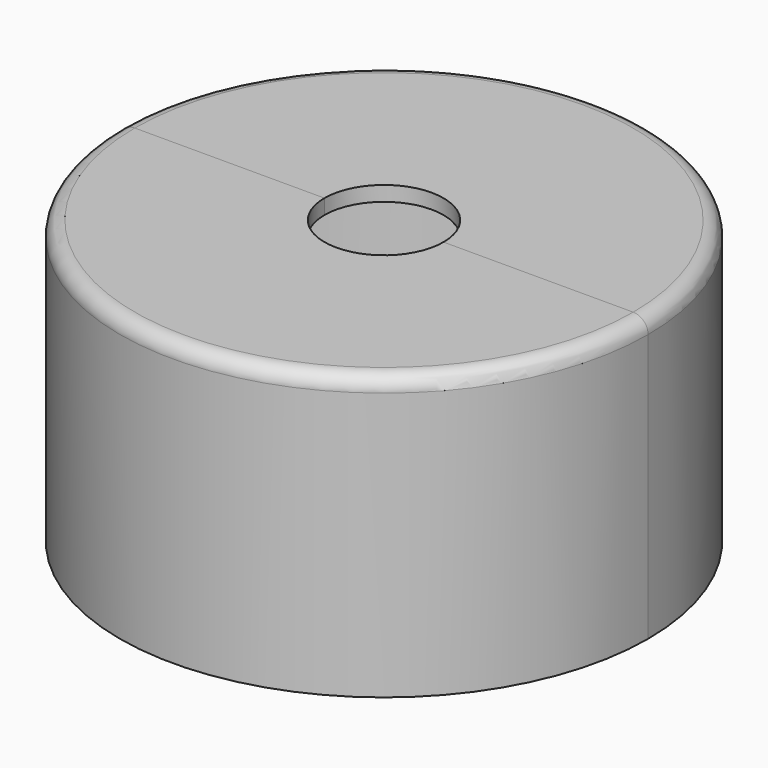
from build123d import *
from build123d import SkipClean  # not in build123d's __all__

# Parameters (mm, degrees)
F3_DEPTH  = 36
F5_DEPTH  = 20
F7_DEPTH  = 36.001
F10_R     = 10
F11_DEPTH = 7
F12_R     = 10
F12_R_2   = 8
F13_DEPTH = 2
F14_W     = 113.5210208595
F14_H     = 51.0865971446
F15_DEPTH = 38.001
F16_W     = 26.7383140922
F16_H     = 24.3122323528
F17_DEPTH = 36
F18_R     = 2
F20_DEPTH = 5


with BuildPart() as f1:
    # F0 (on Front) → F1 (revolve)
    with BuildSketch(Plane.XZ):
        Polygon((26, -5), (27.5, -5), (27.5, 31), (0, 31), (0, 26), (26, 26), (26, 0), align=None)
    revolve(axis=Axis((0, 0, 28.5), (0, 0, 1)))

    # F2 (on face) → F3 (join, through all)
    with BuildSketch(Plane(origin=(0, 0, -5), x_dir=(1, 0, 0), z_dir=(0, 0, -1))):
        with BuildLine():
            Line((-23.5584379788, 11), (23.5584379788, 11))
            ThreePointArc((23.5584379788, 11), (0, 26), (-23.5584379788, 11))
        make_face()
        with BuildLine():
            Line((23.5584379788, -11), (-23.5584379788, -11))
            ThreePointArc((-23.5584379788, -11), (0, -26), (23.5584379788, -11))
        make_face()
    extrude(amount=-F3_DEPTH)

    # F4 (on Front) → F5 (cut, symmetric)
    with BuildSketch(Plane.XZ):
        with BuildLine():
            Line((4.5, -4.6839690926), (3.5, -1.9364916731))
            ThreePointArc((3.5, -1.9364916731), (3.4457195687, 2.0315060063), (0, 4))
            ThreePointArc((0, 4), (-3.4457195687, 2.0315060063), (-3.5, -1.9364916731))
            Line((-3.5, -1.9364916731), (-4.5, -4.6839690926))
            Line((-4.5, -4.6839690926), (-4.5, -5))
            Line((-4.5, -5), (0, -5))
            Line((0, -5), (4.5, -5))
            Line((4.5, -5), (4.5, -4.6839690926))
        make_face()
    extrude(amount=F5_DEPTH, both=True, mode=Mode.SUBTRACT)

    # F6 (on face) → F7 (cut, through all)
    with BuildSketch(Plane(origin=(0, 0, -5), x_dir=(1, 0, 0), z_dir=(0, 0, -1))):
        with BuildLine():
            Line((24.2332416321, -13), (6.5, -13))
            Line((6.5, -13), (6.5, -22))
            Line((6.5, -22), (-6.5, -22))
            Line((-6.5, -22), (-6.5, -13))
            Line((-6.5, -13), (-24.2332416321, -13))
            ThreePointArc((-24.2332416321, -13), (0, -27.5), (24.2332416321, -13))
        make_face()
        with BuildLine():
            Line((6.5, 22), (6.5, 13))
            Line((6.5, 13), (24.2332416321, 13))
            ThreePointArc((24.2332416321, 13), (0, 27.5), (-24.2332416321, 13))
            Line((-24.2332416321, 13), (-6.5, 13))
            Line((-6.5, 13), (-6.5, 22))
            Line((-6.5, 22), (6.5, 22))
        make_face()
    extrude(amount=-F7_DEPTH, mode=Mode.SUBTRACT)

    # F8 (on Front) → F9 (revolve)
    with BuildSketch(Plane.XZ):
        Polygon((26, -5), (27.5, -5), (27.5, 33), (-8, 33), (-8, 31), (26, 31), align=None)
    revolve(axis=Axis((-8, 0, 32), (0, 0, -1)))

    # F10 (on face) → F11 (cut, through all)
    with BuildSketch(Plane.XY.offset(33)):
        with Locations((-8, 0)):
            Circle(F10_R)
    extrude(amount=-F11_DEPTH, mode=Mode.SUBTRACT)

    # F12 (on face) → F13 (join)
    with BuildSketch(Plane.XY.offset(33)):
        with Locations((-8, 0)):
            Circle(F12_R)
        with Locations((-8, 0)):
            Circle(F12_R_2, mode=Mode.SUBTRACT)
    extrude(amount=-F13_DEPTH)

    # F14 (on face) → F15 (cut, through all)
    with BuildSketch(Plane.XY.offset(33)):
        with Locations((0.0438708812, -25.5432985723)):
            Rectangle(F14_W, F14_H)
    extrude(amount=-F15_DEPTH, mode=Mode.SUBTRACT)

    # F16 (on face) → F17 (cut, through all)
    with BuildSketch(Plane(origin=(0, 0, -5), x_dir=(1, 0, 0), z_dir=(0, 0, -1))):
        with Locations((-19.8691570461, -0.8438838236)):
            Rectangle(F16_W, F16_H)
    extrude(amount=-F17_DEPTH, mode=Mode.SUBTRACT)

    # F18
    f18_edges = [f1.edges().sort_by_distance(p)[0] for p in [
        (-14.627107, 33.347885, 31),
        (-8, 35.5, 33),
        (-6.5, 15.94343, 31),
        (0, 22, 31),
        (6.5, 17.5, 31),
        (14.958278, 13, 31),
    ]]
    fillet(f18_edges, radius=F18_R)

    # F19 (on face) → F20 (cut, through all)
    with BuildSketch(Plane(origin=(0, 0, 26), x_dir=(1, 0, 0), z_dir=(0, 0, -1))):
        with BuildLine():
            ThreePointArc((2, 0), (-0.4171245559, -6.5192024052), (-6.5, -9.8868599666))
            Line((-6.5, -9.8868599666), (-6.5, -11))
            Line((-6.5, -11), (23.5584379788, -11))
            ThreePointArc((23.5584379788, -11), (25.3822712483, -5.6338535902), (26, 0))
            Line((26, 0), (2, 0))
        make_face()
    extrude(amount=-F20_DEPTH, mode=Mode.SUBTRACT)

    # F21: F1 across face


with BuildPart() as f1_1:
    add(f1.part, clean=False)
    with SkipClean():  # cleaning this boolean's faces spoils the solid; the shape is the same uncleaned
        add(f1.part.mirror(Plane(origin=(-36.1785540273, 0, 22.5714053698), x_dir=(1, 0, 0), z_dir=(0, -1, 0))), clean=False)


solid = f1_1.part
